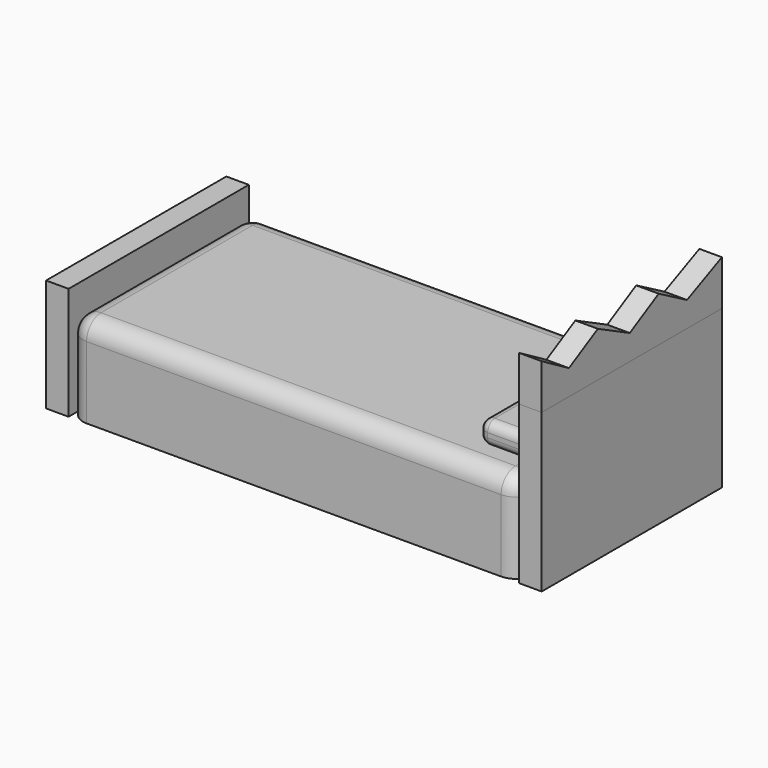
from build123d import *

# Parameters (mm, degrees)
F0_W          = 127
F0_H          = 25.4
F1_DEPTH      = 63.5
F2_R          = 5.08
F3_R          = 5.08
F4_W          = 63.5
F4_H          = 31.75
F5_DEPTH      = 6.35
F6_W          = 63.5
F6_H          = 44.45
F7_DEPTH      = 6.35
F8_W          = 6.35
F8_H          = 63.5
F9_DEPTH      = 12.7
F11_DEPTH     = 25.4
F12_TEXT_SIZE = 12.1132729368
F13_DEPTH     = 0.127
F14_W         = 17.78
F14_H         = 25.4
F15_DEPTH     = 6.35
F16_R         = 2.54
F17_F1_R      = 2.54
F17_F2_R      = 2.54
F17_F3_R      = 2.54
F17_F4_R      = 2.54
F18_R         = 2.54
F19_T1_DEPTH  = 21.59
F19_S5_W      = 2.54
F19_S5_H      = 2.54
F19_T6_DEPTH  = 2.54
F23_DEPTH     = 0.254


# Not quite as in the source:
# - a fillet or chamfer that OpenCascade refuses, or shapes differently, is made with other operations: its cross-section is extruded or revolved along the edge and cut away or added
# - a feature of the source that left no trace in its solid (it failed there, or was rolled back) is left out
# - Text() gives the source's letters only with a copy of the font that has no kerning and outlines rounded to 1/6400 em; it was checked with that copy


with BuildPart() as f1:
    # F0 (on Front) → F1 (new body)
    with BuildSketch(Plane.XZ):
        Rectangle(F0_W, F0_H)
    extrude(amount=F1_DEPTH)

    # F2
    f2_edges = [f1.edges().sort_by_distance(p)[0] for p in [
        (0, -63.5, 12.7),
        (0, 0, 12.7),
    ]]
    fillet(f2_edges, radius=F2_R)

    # F3
    f3_edges = [f1.edges().sort_by_distance(p)[0] for p in [
        (-63.5, -63.5, -2.54),
        (63.5, -63.5, -2.54),
        (-63.5, 0, -2.54),
        (63.5, 0, -2.54),
    ]]
    fillet(f3_edges, radius=F3_R)


with BuildPart() as f5:
    # F4 (on face) → F5 (new body)
    with BuildSketch(Plane(origin=(-63.5, 0, 0), x_dir=(0, -1, 0), z_dir=(-1, 0, 0))):
        with Locations((31.75, 3.175)):
            Rectangle(F4_W, F4_H)
    extrude(amount=F5_DEPTH)


with BuildPart() as f7:
    # F6 (on face) → F7 (new body)
    with BuildSketch(Plane.YZ.offset(63.5)):
        with Locations((-31.75, 9.525)):
            Rectangle(F6_W, F6_H)
    extrude(amount=F7_DEPTH)


with BuildPart() as f9:
    # F8 (on face) → F9 (new body)
    with BuildSketch(Plane.XY.offset(31.75)):
        with Locations((66.675, -31.75)):
            Rectangle(F8_W, F8_H)
    extrude(amount=F9_DEPTH)

    # F10 (on face) → F11 (cut)
    with BuildSketch(Plane(origin=(63.5, 0, 0), x_dir=(0, -1, 0), z_dir=(-1, 0, 0))):
        Polygon((22.2839526832, 44.45), (0, 44.45), (12.3092317954, 38.8377457857), align=None)
        Polygon((63.5, 44.45), (43.7189936638, 44.45), (53.9059452713, 38.8377457857), align=None)
        Polygon((43.7189936638, 44.45), (22.2839526832, 44.45), (32.4709042907, 38.8377457857), align=None)
    extrude(amount=-F11_DEPTH, mode=Mode.SUBTRACT)


with BuildPart() as f13:
    # F12 (on face) → F13 (new body)
    with BuildSketch(Plane(origin=(63.5, 0, 0), x_dir=(0, -1, 0), z_dir=(-1, 0, 0))):
        with Locations((9.1098630801, 21.2617106736)):
            Text('Shelby', F12_TEXT_SIZE, font='Open Sans', font_style=FontStyle.BOLD, text_align=(TextAlign.LEFT, TextAlign.BOTTOM))
    extrude(amount=F13_DEPTH)


with BuildPart() as f15:
    # F14 (on face) → F15 (new body)
    with BuildSketch(Plane.XY.offset(12.7)):
        with Locations((54.6045303345, -15.9758752101)):
            Rectangle(F14_W, F14_H)
    extrude(amount=F15_DEPTH)

    # F16
    f16_edges = [f15.edges().sort_by_distance(p)[0] for p in [
        (45.71453, -15.975875, 19.05),
    ]]
    fillet(f16_edges, radius=F16_R)

    # F17: fillet of radius 2.54 on 5 edges, made by hand

    # F17_f1
    f17_f1_edges = [f15.edges().sort_by_distance(p)[0] for p in [
        (45.7145303345, -3.2758752101, 14.605),
        (46.4584791103, -3.2758752101, 18.3060512242),
        (55.8745303345, -3.2758752101, 19.05),
    ]]
    fillet(f17_f1_edges, radius=F17_F1_R)

    # F17_f2
    f17_f2_edges = [f15.edges().sort_by_distance(p)[0] for p in [
        (45.7145303345, -17.2458752101, 12.7),
    ]]
    fillet(f17_f2_edges, radius=F17_F2_R)

    # F17_f3
    f17_f3_edges = [f15.edges().sort_by_distance(p)[0] for p in [
        (45.7145303345, -28.6758752101, 15.875),
        (46.4584791103, -28.6758752101, 18.3060512242),
        (55.8745303345, -28.6758752101, 19.05),
    ]]
    fillet(f17_f3_edges, radius=F17_F3_R)

    # F17_f4
    f17_f4_edges = [f15.edges().sort_by_distance(p)[0] for p in [
        (63.4945303345, -15.9758752101, 19.05),
    ]]
    fillet(f17_f4_edges, radius=F17_F4_R)


with BuildPart() as f15b:
    # F14 (on face) → F15, piece 2 (new body)
    with BuildSketch(Plane.XY.offset(12.7)):
        with Locations((54.647651329, -42.8917024612)):
            Rectangle(F14_W, F14_H)
    extrude(amount=F15_DEPTH)

    # F18
    f18_edges = [f15b.edges().sort_by_distance(p)[0] for p in [
        (54.647651, -30.191702, 19.05),
        (45.757651, -42.891702, 19.05),
        (54.647651, -55.591702, 19.05),
        (63.537651, -42.891702, 19.05),
        (45.757651, -30.191702, 15.875),
        (45.757651, -42.891702, 12.7),
        (54.647651, -55.591702, 12.7),
        (45.757651, -55.591702, 15.875),
    ]]
    fillet(f18_edges, radius=F18_R)

    # F19: fillet of radius 2.54 on 1 edges, made by hand

    # F19_s2 → F19_t1 (cut)
    with BuildSketch(Plane.YZ.offset(48.297651329)):
        with BuildLine():
            ThreePointArc((-30.1917024612, 15.24), (-30.935651237, 13.4439487758), (-32.7317024612, 12.7))
            Line((-32.7317024612, 12.7), (-30.1917024612, 12.7))
            Line((-30.1917024612, 12.7), (-30.1917024612, 15.24))
        make_face()
    extrude(amount=F19_T1_DEPTH, mode=Mode.SUBTRACT)


with BuildPart() as f19_tool4:
    # F19_s5 → F19_t6 (new body)
    with BuildSketch(Plane.XZ.offset(32.7317024612)):
        with Locations((47.027651329, 13.97)):
            Rectangle(F19_S5_W, F19_S5_H)
    extrude(amount=-F19_T6_DEPTH)

    # F19_s7 → F19_t8 (revolve, cut)
    with BuildSketch(Plane(origin=(48.297651329, -32.7317024612, 15.24), x_dir=(0.7071067812, 0, 0.7071067812), z_dir=(-0.7071067812, 0, 0.7071067812))):
        with BuildLine():
            ThreePointArc((0, -2.54), (2.54, 0), (0, 2.54))
            Line((0, 2.54), (0, -2.54))
        make_face()
    revolve(axis=Axis((48.297651329, -32.7317024612, 15.24), (0, 1, 0)), mode=Mode.SUBTRACT)


with BuildPart() as f15b_1:
    add(f15b.part)

    # F19_t3: cut F19_tool4
    add(f19_tool4.part, mode=Mode.SUBTRACT)


with BuildPart() as f23:
    # F22 (on face) → F23 (new body)
    with BuildSketch(Plane(origin=(-69.85, 0, 0), x_dir=(0, -1, 0), z_dir=(-1, 0, 0))):
        with BuildLine():
            add(Edge.make_bspline(
                [(29.7603625804, 12.5324069522), (27.7605775663, 15.4103248852), (20.5031553482, 17.2992676008), (12.5780952559, 14.2438733524), (8.5014935959, 9.197095017), (9.8218219964, 1.0978513346), (17.5255520568, -5.2265959231), (32.7197676481, -11.271870853), (32.1319070964, -12.4503317707), (47.143751241, -4.3541310123), (53.8034892267, 1.8081688165), (54.5998978958, 8.9976409276), (51.1705641971, 14.180375284), (46.5945002392, 16.3687135662), (40.9090757331, 16.0918133191), (36.652048135, 12.4560376267), (32.7039010311, 8.8657472199), (32.0564352458, 4.7298841497), (31.3821457205, 10.1984766801), (29.7603625804, 12.5324069522)],
                knots=[0, 0, 0, 0, 0.0717143189, 0.1371419539, 0.1921173096, 0.2517804544, 0.3284170915, 0.4164922185, 0.4261133897, 0.5147518546, 0.5887426167, 0.6453531642, 0.7002198905, 0.7505826881, 0.8029282279, 0.8569344912, 0.9110870514, 0.9418412117, 1, 1, 1, 1], degree=3))
        make_face()
    extrude(amount=F23_DEPTH)


solid = Compound([f1.part, f5.part, f7.part, f9.part, f13.part, f15.part, f15b_1.part, f23.part])
